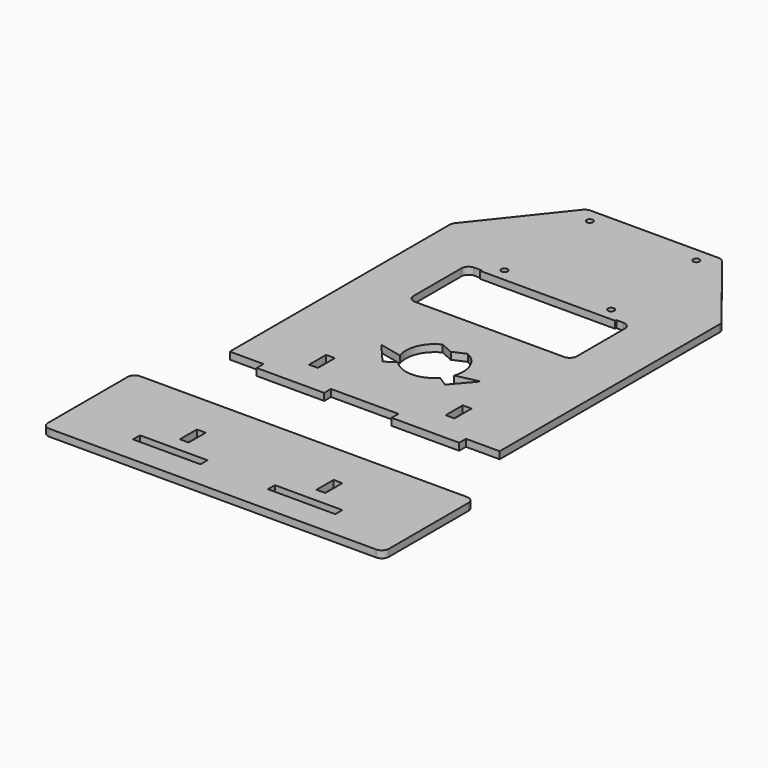
from build123d import *

# Parameters (mm, degrees)
F1_DEPTH = 5


with BuildPart() as f1:
    # F0 (on Top) → F1 (new body)
    with BuildSketch(Plane.XY):
        with BuildLine():
            Line((92.1250784397, -243.4596419334), (-22.8749215603, -243.4596419334))
            Line((-22.8749215603, -243.4596419334), (-137.8749215603, -243.4596419334))
            ThreePointArc((-137.8749215603, -243.4596419334), (-141.4104554662, -244.9241080275), (-142.8749215603, -248.4596419334))
            Line((-142.8749215603, -248.4596419334), (-142.8749215603, -283.4596419334))
            Line((-142.8749215603, -283.4596419334), (-142.8749215603, -298.4596419334))
            Line((-142.8749215603, -298.4596419334), (-142.8749215603, -318.4596419334))
            ThreePointArc((-142.8749215603, -318.4596419334), (-141.4104554662, -321.9951758394), (-137.8749215603, -323.4596419334))
            Line((-137.8749215603, -323.4596419334), (92.1250784397, -323.4596419334))
            ThreePointArc((92.1250784397, -323.4596419334), (95.6606123456, -321.9951758394), (97.1250784397, -318.4596419334))
            Line((97.1250784397, -318.4596419334), (97.1250784397, -248.4596419334))
            ThreePointArc((97.1250784397, -248.4596419334), (95.6606123456, -244.9241080275), (92.1250784397, -243.4596419334))
        make_face()
        Polygon((-94.1249215603, -303.4596419334), (-94.1249215603, -298.4596419334), (-46.6249215603, -298.4596419334), (-46.6249215603, -303.4596419334), (-46.6249215603, -304.6596419334), (-94.1249215603, -304.6596419334), align=None, mode=Mode.SUBTRACT)
        Polygon((-72.8749215603, -273.4596419334), (-70.3749215603, -273.4596419334), (-67.8749215603, -273.4596419334), (-67.8749215603, -288.4596419334), (-72.8749215603, -288.4596419334), (-74.0749215603, -288.4596419334), (-74.0749215603, -273.4596419334), align=None, mode=Mode.SUBTRACT)
        Polygon((0.8750784397, -304.6596419334), (0.8750784397, -303.4596419334), (0.8750784397, -298.4596419334), (48.3750784397, -298.4596419334), (48.3750784397, -303.4596419334), (48.3750784397, -304.6596419334), align=None, mode=Mode.SUBTRACT)
        Polygon((22.1250784397, -273.4596419334), (24.6250784397, -273.4596419334), (27.1250784397, -273.4596419334), (28.3250784397, -273.4596419334), (28.3250784397, -288.4596419334), (27.1250784397, -288.4596419334), (22.1250784397, -288.4596419334), align=None, mode=Mode.SUBTRACT)
    extrude(amount=F1_DEPTH)


with BuildPart() as f1b:
    # F0 (on Top) → F1, piece 2 (new body)
    with BuildSketch(Plane.XY):
        with BuildLine():
            Line((14.6250784397, 65.2551365197), (-60.3749215603, 65.2551365197))
            Line((-60.3749215603, 65.2551365197), (-67.9641170056, 65.2551365197))
            ThreePointArc((-67.9641170056, 65.2551365197), (-70.135678908, 64.758948117), (-71.8762392778, 63.3688640813))
            Line((-71.8762392778, 63.3688640813), (-116.7870438325, 6.9424249383))
            ThreePointArc((-116.7870438325, 6.9424249383), (-117.5951234289, 5.4778469514), (-117.8749215603, 3.8286973767))
            Line((-117.8749215603, 3.8286973767), (-117.8749215603, -52.7448634803))
            Line((-117.8749215603, -52.7448634803), (-117.8749215603, -189.7448634803))
            Line((-117.8749215603, -189.7448634803), (-94.1249215603, -189.7448634803))
            Line((-94.1249215603, -189.7448634803), (-94.1249215603, -194.7448634803))
            Line((-94.1249215603, -194.7448634803), (-94.1249215603, -195.7448634803))
            Line((-94.1249215603, -195.7448634803), (-46.6249215603, -195.7448634803))
            Line((-46.6249215603, -195.7448634803), (-46.6249215603, -194.7448634803))
            Line((-46.6249215603, -194.7448634803), (-46.6249215603, -189.7448634803))
            Line((-46.6249215603, -189.7448634803), (-22.8749215603, -189.7448634803))
            Line((-22.8749215603, -189.7448634803), (0.8750784397, -189.7448634803))
            Line((0.8750784397, -189.7448634803), (0.8750784397, -194.7448634803))
            Line((0.8750784397, -194.7448634803), (0.8750784397, -195.7448634803))
            Line((0.8750784397, -195.7448634803), (48.3750784397, -195.7448634803))
            Line((48.3750784397, -195.7448634803), (48.3750784397, -194.7448634803))
            Line((48.3750784397, -194.7448634803), (48.3750784397, -189.7448634803))
            Line((48.3750784397, -189.7448634803), (72.1250784397, -189.7448634803))
            Line((72.1250784397, -189.7448634803), (72.1250784397, -52.7448634803))
            Line((72.1250784397, -52.7448634803), (72.1250784397, 3.8286973767))
            ThreePointArc((72.1250784397, 3.8286973767), (71.8452803083, 5.4778469514), (71.0372007119, 6.9424249383))
            Line((71.0372007119, 6.9424249383), (26.1263961572, 63.3688640813))
            ThreePointArc((26.1263961572, 63.3688640813), (24.3858357875, 64.758948117), (22.214273885, 65.2551365197))
            Line((22.214273885, 65.2551365197), (14.6250784397, 65.2551365197))
        make_face()
        Polygon((-72.8749215603, -159.7448634803), (-70.3749215603, -159.7448634803), (-67.8749215603, -159.7448634803), (-67.8749215603, -174.7448634803), (-72.8749215603, -174.7448634803), (-74.0749215603, -174.7448634803), (-74.0749215603, -159.7448634803), align=None, mode=Mode.SUBTRACT)
        Polygon((22.1250784397, -159.7448634803), (24.6250784397, -159.7448634803), (27.1250784397, -159.7448634803), (28.3250784397, -159.7448634803), (28.3250784397, -174.7448634803), (27.1250784397, -174.7448634803), (22.1250784397, -174.7448634803), align=None, mode=Mode.SUBTRACT)
        with BuildLine():
            ThreePointArc((-41.9616178547, -134.9464001798), (-41.5936592763, -120.5938582844), (-31.7935436802, -110.1015474486))
            Line((-31.7935436802, -110.1015474486), (-22.8749215603, -114.0089929104))
            Line((-22.8749215603, -114.0089929104), (-13.9562994404, -110.1015474486))
            ThreePointArc((-13.9562994404, -110.1015474486), (-4.1561838443, -120.5938582844), (-3.7882252659, -134.9464001798))
            Line((-3.7882252659, -134.9464001798), (12.1750198305, -131.392210722))
            Line((12.1750198305, -131.392210722), (-0.8886083961, -146.6006189585))
            Line((-0.8886083961, -146.6006189585), (-8.0198945936, -141.9809370457))
            ThreePointArc((-8.0198945936, -141.9809370457), (-22.8749215603, -148.4804743528), (-37.729948527, -141.9809370457))
            Line((-37.729948527, -141.9809370457), (-44.8612347245, -146.6006189585))
            Line((-44.8612347245, -146.6006189585), (-57.924862951, -131.392210722))
            Line((-57.924862951, -131.392210722), (-41.9616178547, -134.9464001798))
        make_face(mode=Mode.SUBTRACT)
        with BuildLine():
            ThreePointArc((-60.3749215603, -17.4948634803), (-58.7839313026, -18.1538732226), (-58.1249215603, -19.7448634803))
            ThreePointArc((-58.1249215603, -19.7448634803), (-61.965911818, -21.3358537379), (-60.3749215603, -17.4948634803))
        make_face(mode=Mode.SUBTRACT)
        with BuildLine():
            ThreePointArc((-60.3749215603, 53.0051365197), (-61.965911818, 56.8461267774), (-58.1249215603, 55.2551365197))
            ThreePointArc((-58.1249215603, 55.2551365197), (-58.7839313026, 53.6641462621), (-60.3749215603, 53.0051365197))
        make_face(mode=Mode.SUBTRACT)
        with BuildLine():
            Line((-80.3749215603, -74.9092054367), (-80.3749215603, -52.7448634803))
            Line((-80.3749215603, -52.7448634803), (-80.3749215603, -32.7448634803))
            ThreePointArc((-80.3749215603, -32.7448634803), (-78.9104554662, -29.2093295743), (-75.3749215603, -27.7448634803))
            Line((-75.3749215603, -27.7448634803), (-70.3749215603, -27.7448634803))
            Line((-70.3749215603, -27.7448634803), (-70.3749215603, -28.7448634803))
            Line((-70.3749215603, -28.7448634803), (24.6250784397, -28.7448634803))
            Line((24.6250784397, -28.7448634803), (24.6250784397, -27.7448634803))
            Line((24.6250784397, -27.7448634803), (29.6250784397, -27.7448634803))
            ThreePointArc((29.6250784397, -27.7448634803), (33.1606123456, -29.2093295743), (34.6250784397, -32.7448634803))
            Line((34.6250784397, -32.7448634803), (34.6250784397, -74.9092054367))
            ThreePointArc((34.6250784397, -74.9092054367), (33.1606123456, -78.4447393426), (29.6250784397, -79.9092054367))
            Line((29.6250784397, -79.9092054367), (-75.3749215603, -79.9092054367))
            ThreePointArc((-75.3749215603, -79.9092054367), (-78.9104554662, -78.4447393426), (-80.3749215603, -74.9092054367))
        make_face(mode=Mode.SUBTRACT)
        with BuildLine():
            ThreePointArc((14.6250784397, -17.4948634803), (16.2160686974, -18.1538732226), (16.8750784397, -19.7448634803))
            ThreePointArc((16.8750784397, -19.7448634803), (14.6250784397, -21.9948634803), (12.3750784397, -19.7448634803))
            ThreePointArc((12.3750784397, -19.7448634803), (13.034088182, -18.1538732226), (14.6250784397, -17.4948634803))
        make_face(mode=Mode.SUBTRACT)
        with BuildLine():
            ThreePointArc((16.8750784397, 55.2551365197), (16.2160686974, 53.6641462621), (14.6250784397, 53.0051365197))
            ThreePointArc((14.6250784397, 53.0051365197), (13.034088182, 53.6641462621), (12.3750784397, 55.2551365197))
            ThreePointArc((12.3750784397, 55.2551365197), (14.6250784397, 57.5051365197), (16.8750784397, 55.2551365197))
        make_face(mode=Mode.SUBTRACT)
    extrude(amount=F1_DEPTH)


solid = Compound([f1.part, f1b.part])
